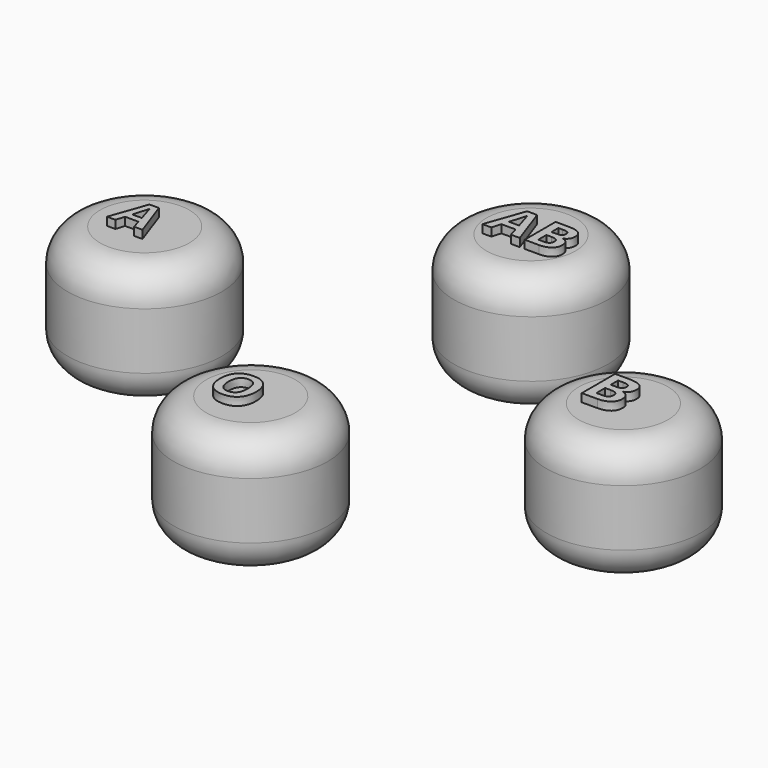
from build123d import *

# Parameters (mm, degrees)
F0_R         = 12.065
F1_DEPTH     = 19.05
F2_R         = 5.08
F2_2_R       = 5.08
F2_3_R       = 5.08
F2_4_R       = 5.08
F3_TEXT_SIZE = 8.0555884375
F4_DEPTH     = 1.27
F5_TEXT_SIZE = 8.4795601045
F6_DEPTH     = 1.27
F7_TEXT_SIZE = 8.3192613804
F8_DEPTH     = 1.27
F9_TEXT_SIZE = 9.1507190114
F10_DEPTH    = 1.27


# Not quite as in the source:
# - Text() gives the source's letters only with a copy of the font that has no kerning and outlines rounded to 1/6400 em; it was checked with that copy


with BuildPart() as f1:
    # F0 (on Top) → F1 (new body)
    with BuildSketch(Plane.XY):
        with Locations((0, -27.0026181623)):
            Circle(F0_R)
    extrude(amount=F1_DEPTH)

    # F2#4
    f2_4_edges = [f1.edges().sort_by_distance(p)[0] for p in [
        (-12.065, -27.002618, 19.05),
        (-12.065, -27.002618, 0),
    ]]
    fillet(f2_4_edges, radius=F2_4_R)

    # F7 (on face) → F8 (join)
    with BuildSketch(Plane.XY.offset(19.05)):
        with Locations((-4.8265182413, -30.5597931147)):
            Text('O', F7_TEXT_SIZE, font='Open Sans', font_style=FontStyle.BOLD, text_align=(TextAlign.LEFT, TextAlign.BOTTOM))
    extrude(amount=F8_DEPTH)


with BuildPart() as f1b:
    # F0 (on Top) → F1, piece 2 (new body)
    with BuildSketch(Plane.XY):
        with Locations((36.7695236325, 0)):
            Circle(F0_R)
    extrude(amount=F1_DEPTH)

    # F2#3
    f2_3_edges = [f1b.edges().sort_by_distance(p)[0] for p in [
        (24.704524, 0, 19.05),
        (24.704524, 0, 0),
    ]]
    fillet(f2_3_edges, radius=F2_3_R)

    # F9 (on face) → F10 (join)
    with BuildSketch(Plane.XY.offset(19.05)):
        with Locations((31.7991226912, -2.9786278028)):
            Text('B', F9_TEXT_SIZE, font='Open Sans', font_style=FontStyle.BOLD, text_align=(TextAlign.LEFT, TextAlign.BOTTOM))
    extrude(amount=F10_DEPTH)


with BuildPart() as f1c:
    # F0 (on Top) → F1, piece 3 (new body)
    with BuildSketch(Plane.XY):
        with Locations((0, 27.8644026815)):
            Circle(F0_R)
    extrude(amount=F1_DEPTH)

    # F2#2
    f2_2_edges = [f1c.edges().sort_by_distance(p)[0] for p in [
        (-12.065, 27.864403, 19.05),
        (-12.065, 27.864403, 0),
    ]]
    fillet(f2_2_edges, radius=F2_2_R)

    # F5 (on face) → F6 (join)
    with BuildSketch(Plane.XY.offset(19.05)):
        with Locations((-4.8236739822, 24.385035038)):
            Text('AB', F5_TEXT_SIZE, font='Open Sans', font_style=FontStyle.BOLD, text_align=(TextAlign.LEFT, TextAlign.BOTTOM))
    extrude(amount=F6_DEPTH)


with BuildPart() as f1d:
    # F0 (on Top) → F1, piece 4 (new body)
    with BuildSketch(Plane.XY):
        with Locations((-38.2058317841, 0)):
            Circle(F0_R)
    extrude(amount=F1_DEPTH)

    # F2
    f2_edges = [f1d.edges().sort_by_distance(p)[0] for p in [
        (-50.270832, 0, 19.05),
        (-50.270832, 0, 0),
    ]]
    fillet(f2_edges, radius=F2_R)

    # F3 (on face) → F4 (join)
    with BuildSketch(Plane.XY.offset(19.05)):
        with Locations((-41.9087074697, -2.7604755014)):
            Text('A', F3_TEXT_SIZE, font='Open Sans', font_style=FontStyle.BOLD, text_align=(TextAlign.LEFT, TextAlign.BOTTOM))
    extrude(amount=F4_DEPTH)


solid = Compound([f1.part, f1b.part, f1c.part, f1d.part])
